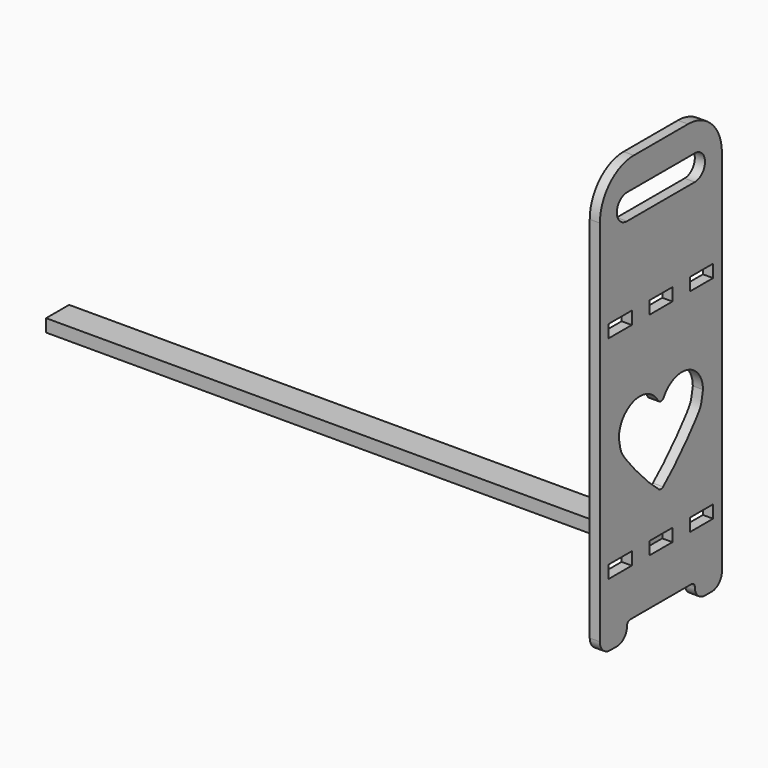
from build123d import *

# Parameters (mm, degrees)
F0_W     = 34
F0_H     = 15
F1_DEPTH = 12
F2_W     = 34
F2_H     = 15
F3_DEPTH = 700


with BuildPart() as f1:
    # F0 (on Right) → F1 (new body)
    with BuildSketch(Plane.YZ):
        with BuildLine():
            Line((0, 452.0943418145), (-40, 452.0943418145))
            ThreePointArc((-40, 452.0943418145), (-75.3553390593, 437.4496808738), (-90, 402.0943418145))
            Line((-90, 402.0943418145), (-90, -32.9056581855))
            ThreePointArc((-90, -32.9056581855), (-85.6066017178, -43.5122599033), (-75, -47.9056581855))
            Line((-75, -47.9056581855), (-65, -47.9056581855))
            ThreePointArc((-65, -47.9056581855), (-54.3933982822, -43.5122599033), (-50, -32.9056581855))
            ThreePointArc((-50, -32.9056581855), (-48.5355339059, -29.3701242795), (-45, -27.9056581855))
            Line((-45, -27.9056581855), (45, -27.9056581855))
            ThreePointArc((45, -27.9056581855), (48.5355339059, -29.3701242795), (50, -32.9056581855))
            ThreePointArc((50, -32.9056581855), (54.3933982822, -43.5122599033), (65, -47.9056581855))
            Line((65, -47.9056581855), (75, -47.9056581855))
            ThreePointArc((75, -47.9056581855), (85.6066017178, -43.5122599033), (90, -32.9056581855))
            Line((90, -32.9056581855), (90, 402.0943418145))
            ThreePointArc((90, 402.0943418145), (75.3553390593, 437.4496808738), (40, 452.0943418145))
            Line((40, 452.0943418145), (0, 452.0943418145))
        make_face()
        with Locations((-60, 34.5943418145)):
            Rectangle(F0_W, F0_H, mode=Mode.SUBTRACT)
        with Locations((0, 34.5943418145)):
            Rectangle(F0_W, F0_H, mode=Mode.SUBTRACT)
        with Locations((60, 34.5943418145)):
            Rectangle(F0_W, F0_H, mode=Mode.SUBTRACT)
        with BuildLine():
            ThreePointArc((4.3057986639, 182.9335873252), (39.183716083, 197.0856083174), (62.0252142978, 167.1688106786))
            add(Edge.make_bspline(
                [(3.1446835541, 90.2015406127), (22.3537729205, 105.7410613962), (58.6775915843, 147.6474664313), (59.6779100597, 153.4350961447), (62.0252142978, 167.1688106786)],
                knots=[0.0335863635, 0.0335863635, 0.0335863635, 0.0335863635, 0.6420190055, 1, 1, 1, 1], degree=3))
            add(Edge.make_bspline(
                [(0, 87.7314905125), (1.0350959007, 88.5189757858), (2.0843139865, 89.3437365482), (3.1446835541, 90.2015406127)],
                knots=[0, 0, 0, 0, 0.0335863635, 0.0335863635, 0.0335863635, 0.0335863635], degree=3))
            add(Edge.make_bspline(
                [(0, 87.7314905125), (-1.0350959007, 88.5189757858), (-2.0843139865, 89.3437365482), (-3.1446835541, 90.2015406127)],
                knots=[0, 0, 0, 0, 0.0335863635, 0.0335863635, 0.0335863635, 0.0335863635], degree=3))
            add(Edge.make_bspline(
                [(-3.1446835541, 90.2015406127), (-22.3537729205, 105.7410613962), (-58.6775915843, 147.6474664313), (-59.6779100597, 153.4350961447), (-62.0252142978, 167.1688106786)],
                knots=[0.0335863635, 0.0335863635, 0.0335863635, 0.0335863635, 0.6420190055, 1, 1, 1, 1], degree=3))
            ThreePointArc((-62.0252142978, 167.1688106786), (-39.183716083, 197.0856083174), (-4.3057986639, 182.9335873252))
            ThreePointArc((-4.3057986639, 182.9335873252), (0, 180.475259583), (4.3057986639, 182.9335873252))
        make_face(mode=Mode.SUBTRACT)
        with Locations((-60, 284.5943418145)):
            Rectangle(F0_W, F0_H, mode=Mode.SUBTRACT)
        with Locations((0, 284.5943418145)):
            Rectangle(F0_W, F0_H, mode=Mode.SUBTRACT)
        with Locations((60, 284.5943418145)):
            Rectangle(F0_W, F0_H, mode=Mode.SUBTRACT)
        with BuildLine():
            Line((-50, 417.7838551998), (0, 417.7838551998))
            Line((0, 417.7838551998), (50, 417.7838551998))
            ThreePointArc((50, 417.7838551998), (60.6066017178, 413.3904569176), (65, 402.7838551998))
            ThreePointArc((65, 402.7838551998), (60.6066017178, 392.177253482), (50, 387.7838551998))
            Line((50, 387.7838551998), (-50, 387.7838551998))
            ThreePointArc((-50, 387.7838551998), (-60.6066017178, 392.177253482), (-65, 402.7838551998))
            ThreePointArc((-65, 402.7838551998), (-60.6066017178, 413.3904569176), (-50, 417.7838551998))
        make_face(mode=Mode.SUBTRACT)
        with BuildLine():
            add(Edge.make_bspline(
                [(0, 87.7314905125), (1.0350959007, 88.5189757858), (2.0843139865, 89.3437365482), (3.1446835541, 90.2015406127)],
                knots=[0, 0, 0, 0, 0.0335863635, 0.0335863635, 0.0335863635, 0.0335863635], degree=3))
            ThreePointArc((3.1446835541, 90.2015406127), (0, 89.0888231268), (-3.1446835541, 90.2015406127))
            add(Edge.make_bspline(
                [(0, 87.7314905125), (-1.0350959007, 88.5189757858), (-2.0843139865, 89.3437365482), (-3.1446835541, 90.2015406127)],
                knots=[0, 0, 0, 0, 0.0335863635, 0.0335863635, 0.0335863635, 0.0335863635], degree=3))
        make_face()
    extrude(amount=F1_DEPTH)


with BuildPart() as f3:
    # F2 (on face) → F3 (new body)
    with BuildSketch(Plane(origin=(0, 0, 0), x_dir=(0, -1, 0), z_dir=(-1, 0, 0))):
        with Locations((0, 34.5943418145)):
            Rectangle(F2_W, F2_H)
    extrude(amount=F3_DEPTH)


solid = Compound([f1.part, f3.part])
